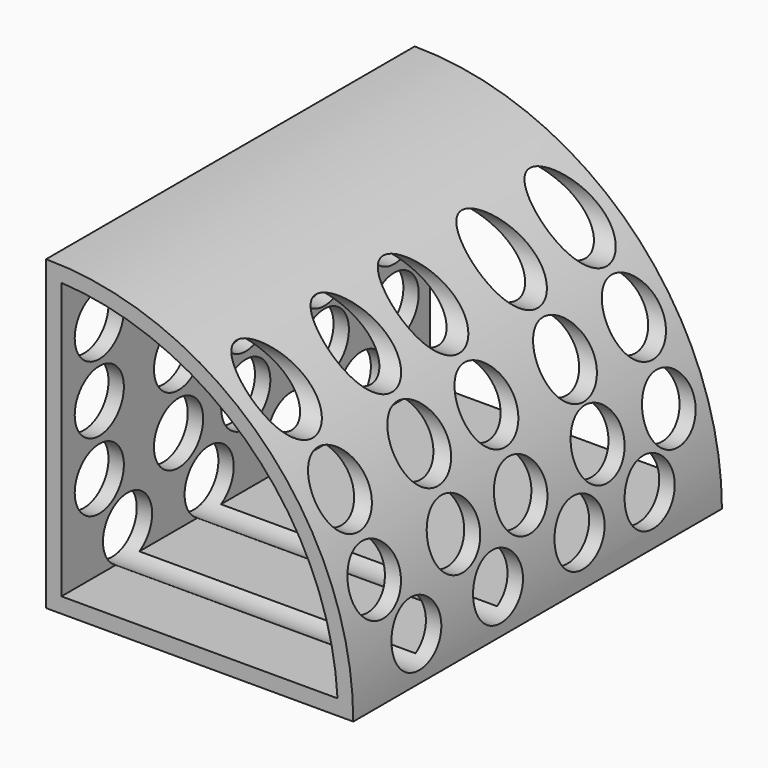
from build123d import *

# Parameters (mm, degrees)
F1_DEPTH = 38.1
F2_T     = -2.54
F4_D     = 10.16


# Not quite as in the source:
# - a feature names something its author has since deleted; it is built from what else it names


with BuildPart() as f1:
    # F0 (on Front) → F1 (new body, symmetric)
    with BuildSketch(Plane.XZ):
        with BuildLine():
            Line((0, 50.8), (0, 0))
            Line((0, 0), (50.8, 0))
            ThreePointArc((50.8, 0), (35.9210244843, 35.9210244843), (0, 50.8))
        make_face()
    extrude(amount=F1_DEPTH, both=True)

    # F2
    f2_openings = [f1.faces().sort_by_distance(p)[0] for p in [
        (21.56019, -38.1, 21.56019),
        (21.56019, 38.1, 21.56019),
    ]]
    offset(amount=F2_T, openings=f2_openings)

    # F4 (through all)
    with Locations(Plane(origin=(0, 0, 0), x_dir=(0, 1, 0), z_dir=(-1, 0, 0))):
        with Locations((30.6795034558, -39.1556384663), (16.2395443767, -38.9857683331), (0, -38.9857683331), (-13.8899311423, -38.9857683331), (-30.2751362324, -38.9857683331), (-30.2751362324, -27.8047341853), (-13.8899311423, -27.8047341853), (16.2395443767, -27.8047341853), (30.6795034558, -28.0428249389), (30.6795034558, -16.6145674884), (16.2395443767, -17.237322405), (0, -16.4841338992), (0, -27.8047341853), (-13.8899311423, -16.4841338992), (-30.2751362324, -16.4841338992), (23.9536166191, -7.8977867961), (9.4604119658, -7.8977867961), (-7.5627407059, -6.9939610548), (-24.4352463633, -6.9939610548)):
            Hole(F4_D / 2)


solid = f1.part
